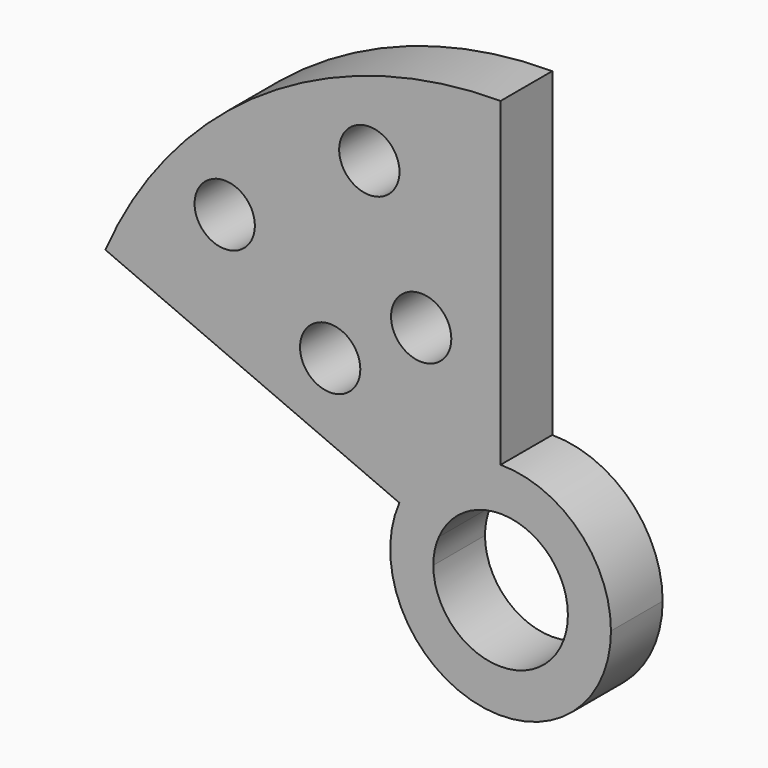
from build123d import *

# Parameters (mm, degrees)
F0_R     = 1.4
F1_DEPTH = 3


# Not quite as in the source:
# - a feature names something its author has since deleted; it is built from what else it names


with BuildPart() as f1:
    # F0 (on Front) → F1 (new body)
    with BuildSketch(Plane.XZ):
        with BuildLine():
            Line((-5.125, 0), (-3.125, 0))
            ThreePointArc((-3.125, 0), (-3.0593081858, 0.6373840479), (-2.8649946083, 1.2479707105))
            Line((-2.8649946083, 1.2479707105), (-4.700755545, 2.0416959387))
            ThreePointArc((-4.700755545, 2.0416959387), (-5.0178181099, 1.0426535455), (-5.125, 0))
        make_face()
        with BuildLine():
            ThreePointArc((3.125, 0), (0, -3.125), (-3.125, 0))
            Line((-3.125, 0), (-5.125, 0))
            ThreePointArc((-5.125, 0), (0, -5.125), (5.125, 0))
            ThreePointArc((5.125, 0), (3.6239222536, 3.6239222536), (0, 5.125))
            Line((0, 5.125), (0, 3.125))
            ThreePointArc((0, 3.125), (2.2097086912, 2.2097086912), (3.125, 0))
        make_face()
        with BuildLine():
            Line((-4.700755545, 2.0416959387), (-2.8649946083, 1.2479707105))
            ThreePointArc((-2.8649946083, 1.2479707105), (-1.7125589814, 2.6139561464), (0, 3.125))
            Line((0, 3.125), (0, 5.125))
            ThreePointArc((0, 5.125), (-2.8108658198, 4.2854006047), (-4.700755545, 2.0416959387))
        make_face()
        with BuildLine():
            Line((-18.3542016569, 7.9450161447), (-4.700755545, 2.0416959387))
            ThreePointArc((-4.700755545, 2.0416959387), (-2.8108658198, 4.2854006047), (0, 5.125))
            Line((0, 5.125), (0, 20))
            ThreePointArc((0, 20), (-10.9795190493, 16.7167628878), (-18.3542016569, 7.9450161447))
        make_face()
        with Locations((-7.9143406, 6.9087709696)):
            Circle(F0_R, mode=Mode.SUBTRACT)
        with Locations((-3.6882084925, 9.5327961412)):
            Circle(F0_R, mode=Mode.SUBTRACT)
        with Locations((-12.8110766731, 11.1833441447)):
            Circle(F0_R, mode=Mode.SUBTRACT)
        with Locations((-6.0959799545, 15.5703980315)):
            Circle(F0_R, mode=Mode.SUBTRACT)
    extrude(amount=F1_DEPTH)


solid = f1.part
